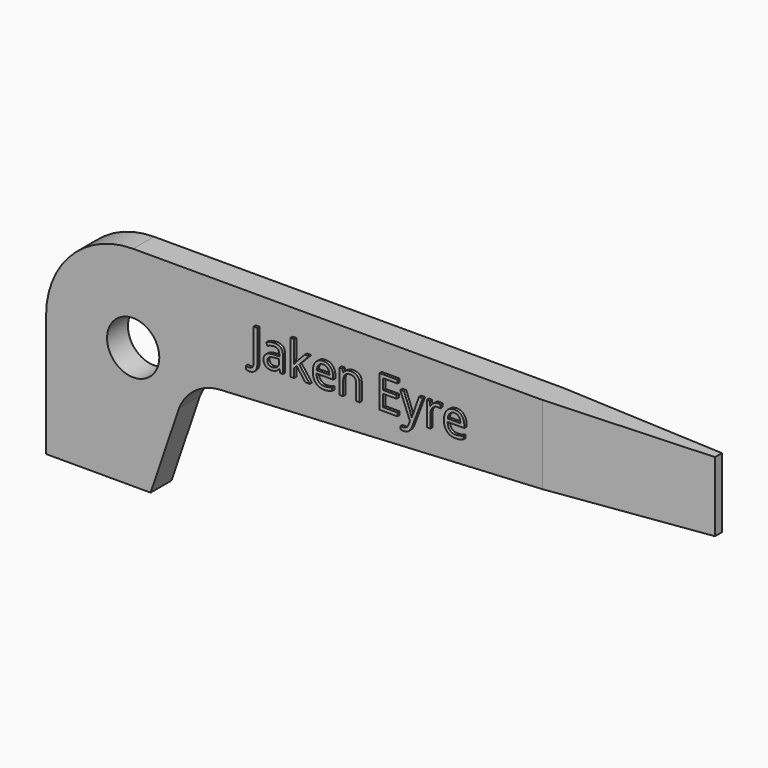
from build123d import *

# Parameters (mm, degrees)
F1_DEPTH     = 2.38125
F2_R         = 2.38125
F3_DEPTH     = 2.38225
F5_DEPTH     = 25.4
F6_TEXT_SIZE = 4.1159322589
F7_DEPTH     = 0.254


# Not quite as in the source:
# - Text() gives the source's letters only with a copy of the font that has no kerning and outlines rounded to 1/6400 em; it was checked with that copy


with BuildPart() as f1:
    # F0 (on Front) → F1 (new body)
    with BuildSketch(Plane.XZ):
        with BuildLine():
            Line((60.325, 19.05), (7.9375, 19.05))
            ThreePointArc((7.9375, 19.05), (2.3248399243, 16.7251600757), (0, 11.1125))
            Line((0, 11.1125), (0, 0))
            Line((0, 0), (9.525, 0))
            Line((9.525, 0), (12.1173647876, 7.6271664624))
            ThreePointArc((12.1173647876, 7.6271664624), (13.6033153977, 9.5214275013), (15.875, 10.31875))
            Line((15.875, 10.31875), (60.325, 12.7))
            Line((60.325, 12.7), (60.325, 19.05))
        make_face()
    extrude(amount=F1_DEPTH)

    # F2 (on face) → F3 (cut, through all)
    with BuildSketch(Plane.XZ.offset(2.38125)):
        with Locations((7.9375, 11.1125)):
            Circle(F2_R)
    extrude(amount=-F3_DEPTH, mode=Mode.SUBTRACT)

    # F4 (on face) → F5 (cut)
    with BuildSketch(Plane.XY.offset(19.05)):
        Polygon((60.325, -2.38125), (60.325, -1.5875), (45.24375, -2.38125), align=None)
        Polygon((60.325, 0), (45.24375, 0), (60.325, -0.79375), align=None)
    extrude(amount=-F5_DEPTH, mode=Mode.SUBTRACT)

    # F6 (on face) → F7 (join)
    with BuildSketch(Plane.XZ.offset(2.38125)):
        with Locations((18.7300425023, 13.6060873047)):
            Text('Jaken Eyre', F6_TEXT_SIZE, font='Open Sans', text_align=(TextAlign.LEFT, TextAlign.BOTTOM))
    extrude(amount=F7_DEPTH)


solid = f1.part
